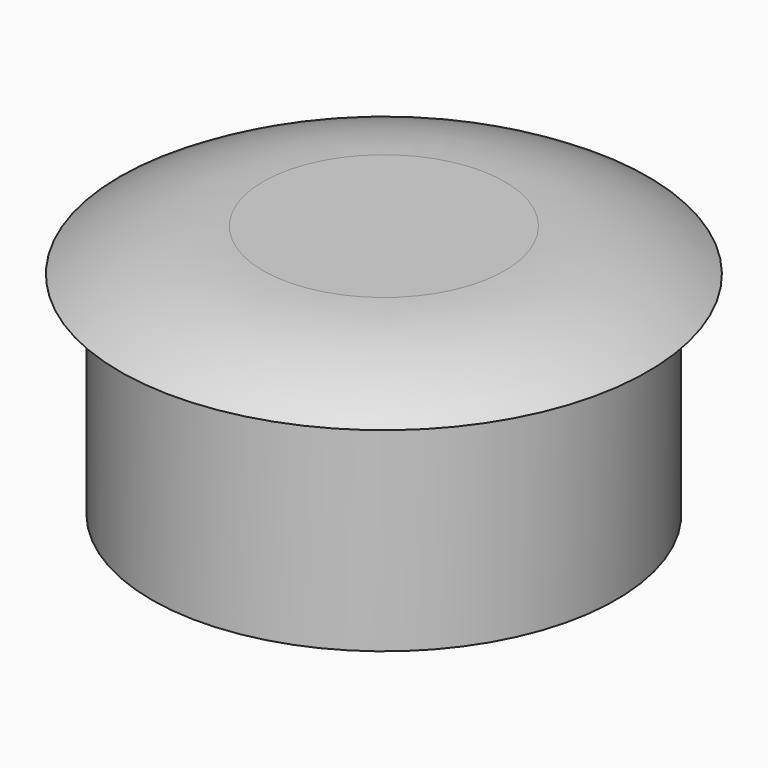
from build123d import *


# Not quite as in the source:
# - a fillet or chamfer that OpenCascade refuses, or shapes differently, is made with other operations: its cross-section is extruded or revolved along the edge and cut away or added


with BuildPart() as f1:
    # F0 (on Front) → F1 (revolve)
    with BuildSketch(Plane.XZ):
        Polygon((0, 7.2039468596), (0, 10.2039468596), (-12.5, 10.2039468596), (-12.5, 8.2039468596), (-11, 8.2039468596), (-11, -1.7960531404), (-9, -1.853223308), (-9, 7.2039468596), align=None)
    revolve(axis=Axis((0, 0, 8.7039468596), (0, 0, -1)))

    # F2: fillet of radius 12.5 on 1 edges, made by hand

    # F2_s1 → F2_t2 (revolve, cut)
    with BuildSketch(Plane.XZ):
        with BuildLine():
            ThreePointArc((-5.7176700169, 10.2039468596), (-9.2532039228, 9.6935256679), (-12.5, 8.2039468596))
            Line((-12.5, 8.2039468596), (-12.6356465997, 8.4139468596))
            ThreePointArc((-12.6356465997, 8.4139468596), (-12.75, 9.2039468596), (-12.75, 10.2039468596))
            Line((-12.75, 10.2039468596), (-12.5, 10.4539468596))
            Line((-12.5, 10.4539468596), (-5.7176700169, 10.4539468596))
            Line((-5.7176700169, 10.4539468596), (-5.7176700169, 10.2039468596))
        make_face()
    revolve(axis=Axis((0, 0, 10.2039468596), (0, 0, -1)), mode=Mode.SUBTRACT)


solid = f1.part
